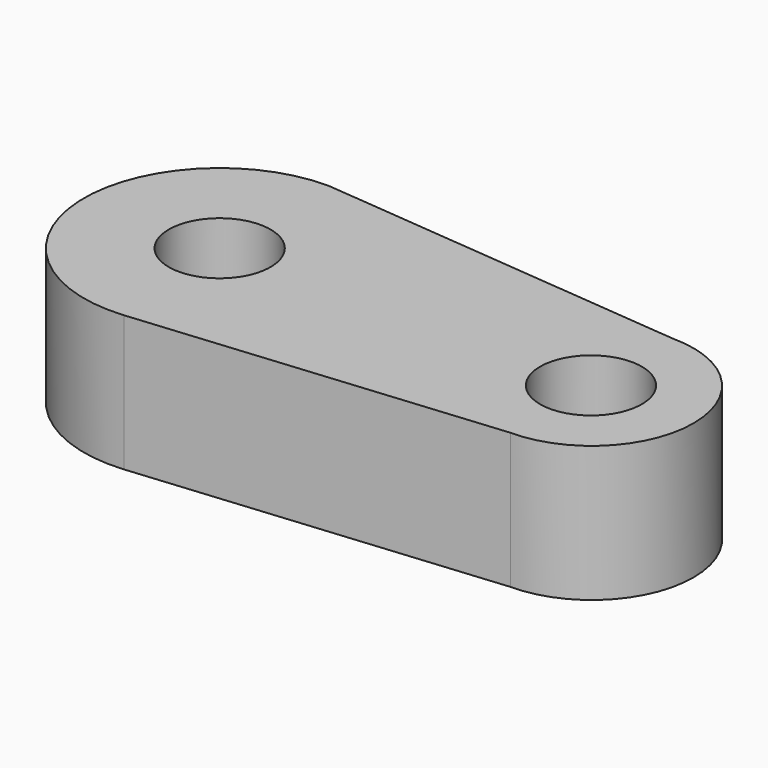
from build123d import *

# Parameters (mm, degrees)
F2_DEPTH = 25.4
F3_D     = 19.05
F3_DEPTH = 25.4
F3_TIP   = 5.7231973962


with BuildPart() as f2:
    # F0 (on Top) → F2 (new body)
    with BuildSketch(Plane.XY):
        with BuildLine():
            ThreePointArc((2.3458816171, -25.2914380658), (18.7715928077, -17.1110287085), (25.4, 0))
            ThreePointArc((25.4, 0), (19.5173228231, 16.2552794445), (4.5941645813, 24.981065866))
            Line((4.5941645813, 24.981065866), (0, 25.4))
            ThreePointArc((0, 25.4), (-25.3728450008, -1.1741961351), (2.3458816171, -25.2914380658))
        make_face()
        with BuildLine():
            ThreePointArc((4.5941645813, 24.981065866), (19.5173228231, 16.2552794445), (25.4, 0))
            ThreePointArc((25.4, 0), (18.7715928077, -17.1110287085), (2.3458816171, -25.2914380658))
            Line((2.3458816171, -25.2914380658), (69.6361139417, -19.05))
            ThreePointArc((69.6361139417, -19.05), (50.5861139417, 0), (69.6361139417, 19.05))
            Line((69.6361139417, 19.05), (4.5941645813, 24.981065866))
        make_face()
        with BuildLine():
            ThreePointArc((88.6861139417, 0), (83.1064981233, 13.4703841816), (69.6361139417, 19.05))
            ThreePointArc((69.6361139417, 19.05), (50.5861139417, 0), (69.6361139417, -19.05))
            ThreePointArc((69.6361139417, -19.05), (83.1064981233, -13.4703841816), (88.6861139417, 0))
        make_face()
    extrude(amount=F2_DEPTH)

    # F3
    with Locations(Plane(origin=(0, 0, 0), x_dir=(1, 0, 0), z_dir=(0, 0, -1))):
        with Locations((0, 0), (69.4895982742, 0)):
            Hole(F3_D / 2, depth=F3_DEPTH)
            with Locations((0, 0, -(F3_DEPTH + F3_TIP / 2))):  # 118° drill point
                Cone(0, F3_D / 2, F3_TIP, mode=Mode.SUBTRACT)


solid = f2.part
